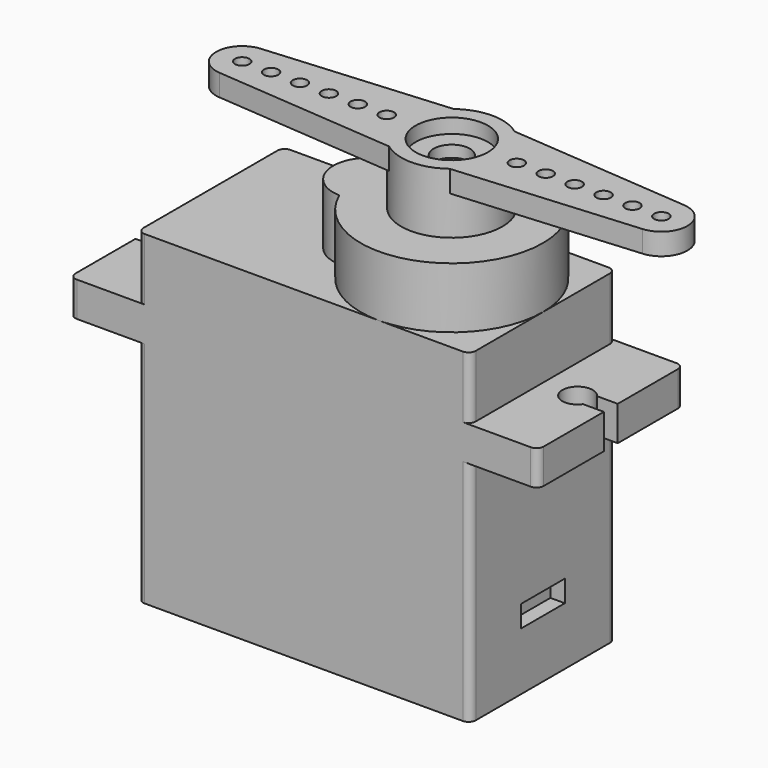
from build123d import *

# Parameters (mm, degrees)
F0_W      = 4.7
F0_H      = 2.4
F1_DEPTH  = 12.6
F3_DEPTH  = 4.2
F4_R      = 2.3
F4_R_2    = 0.9
F5_DEPTH  = 2.5
F7_DEPTH  = 25
F8_R      = 0.5
F9_W      = 3.8
F9_H      = 1.5
F10_DEPTH = 1
F12_R     = 0.5
F13_DEPTH = 1.5
F14_R     = 3.5
F15_DEPTH = 2.7
F16_R     = 2.25
F17_DEPTH = 2.4
F18_R     = 2.5
F19_DEPTH = 1
F20_R     = 1.25
F21_DEPTH = 25


with BuildPart() as f1:
    # F0 (on Front) → F1 (new body)
    with BuildSketch(Plane.XZ):
        Polygon((0, 15.8), (0, 0), (23, 0), (23, 15.8), (23, 18.2), (23, 22.5), (0, 22.5), (0, 18.2), align=None)
        with Locations((-2.35, 17)):
            Rectangle(F0_W, F0_H)
        with Locations((25.35, 17)):
            Rectangle(F0_W, F0_H)
    extrude(amount=F1_DEPTH)

    # F2 (on face) → F3 (join)
    with BuildSketch(Plane.XY.offset(22.5)):
        with BuildLine():
            ThreePointArc((10.9166666667, -3.8013892749), (8.5, -6.3), (10.9166666667, -8.7986107251))
            ThreePointArc((10.9166666667, -8.7986107251), (23, -6.3), (10.9166666667, -3.8013892749))
        make_face()
    extrude(amount=F3_DEPTH)

    # F4 (on face) → F5 (join)
    with BuildSketch(Plane.XY.offset(26.7)):
        with Locations((16.7, -6.3)):
            Circle(F4_R)
        with Locations((16.7, -6.3)):
            Circle(F4_R_2, mode=Mode.SUBTRACT)
    extrude(amount=F5_DEPTH)

    # F6 (on face) → F7 (cut)
    with BuildSketch(Plane.XY.offset(18.2)):
        with BuildLine():
            Line((-5.3876070306, -6.9), (-3.261684397, -6.9))
            ThreePointArc((-3.261684397, -6.9), (-1.35, -6.3), (-3.261684397, -5.7))
            Line((-3.261684397, -5.7), (-5.3876070306, -5.7))
            Line((-5.3876070306, -5.7), (-5.3876070306, -6.9))
        make_face()
        with BuildLine():
            ThreePointArc((26.261684397, -5.7), (24.35, -6.3), (26.261684397, -6.9))
            Line((26.261684397, -6.9), (28.3876070306, -6.9))
            Line((28.3876070306, -6.9), (28.3876070306, -5.7))
            Line((28.3876070306, -5.7), (26.261684397, -5.7))
        make_face()
    extrude(amount=-F7_DEPTH, mode=Mode.SUBTRACT)

    # F8
    f8_edges = [f1.edges().sort_by_distance(p)[0] for p in [
        (0, -12.6, 20.35),
        (0, -12.6, 7.9),
        (0, 0, 20.35),
        (0, 0, 7.9),
        (-4.7, -12.6, 17),
        (-4.7, 0, 17),
        (27.7, -12.6, 17),
        (23, -12.6, 20.35),
        (23, -12.6, 7.9),
        (27.7, 0, 17),
        (23, 0, 20.35),
        (23, 0, 7.9),
    ]]
    fillet(f8_edges, radius=F8_R)

    # F9 (on face) → F10 (cut)
    with BuildSketch(Plane.YZ.offset(23)):
        with Locations((-6.3, 4.75)):
            Rectangle(F9_W, F9_H)
    extrude(amount=-F10_DEPTH, mode=Mode.SUBTRACT)


with BuildPart() as f13:
    # F12 (on offset) → F13 (new body)
    with BuildSketch(Plane(origin=(0, 0, 31), x_dir=(1, 0, 0), z_dir=(0, 0, -1))):
        with BuildLine():
            Line((2.0561389261, 4.5057581012), (14.6, 3.5))
            ThreePointArc((14.6, 3.5), (16.7, 2.8), (18.8, 3.5))
            Line((18.8, 3.5), (31.3438610739, 4.5057581012))
            ThreePointArc((31.3438610739, 4.5057581012), (33, 6.3), (31.3438610739, 8.0942418988))
            Line((31.3438610739, 8.0942418988), (18.8, 9.1))
            ThreePointArc((18.8, 9.1), (16.7, 9.8), (14.6, 9.1))
            Line((14.6, 9.1), (2.0561389261, 8.0942418988))
            ThreePointArc((2.0561389261, 8.0942418988), (0.4, 6.3), (2.0561389261, 4.5057581012))
        make_face()
        with Locations((2.2, 6.3)):
            Circle(F12_R, mode=Mode.SUBTRACT)
        with Locations((4.2, 6.3)):
            Circle(F12_R, mode=Mode.SUBTRACT)
        with Locations((6.2, 6.3)):
            Circle(F12_R, mode=Mode.SUBTRACT)
        with Locations((8.2, 6.3)):
            Circle(F12_R, mode=Mode.SUBTRACT)
        with Locations((10.2, 6.3)):
            Circle(F12_R, mode=Mode.SUBTRACT)
        with Locations((12.2, 6.3)):
            Circle(F12_R, mode=Mode.SUBTRACT)
        with Locations((21.2, 6.3)):
            Circle(F12_R, mode=Mode.SUBTRACT)
        with Locations((23.2, 6.3)):
            Circle(F12_R, mode=Mode.SUBTRACT)
        with Locations((25.2, 6.3)):
            Circle(F12_R, mode=Mode.SUBTRACT)
        with Locations((27.2, 6.3)):
            Circle(F12_R, mode=Mode.SUBTRACT)
        with Locations((29.2, 6.3)):
            Circle(F12_R, mode=Mode.SUBTRACT)
        with Locations((31.2, 6.3)):
            Circle(F12_R, mode=Mode.SUBTRACT)
    extrude(amount=F13_DEPTH)

    # F14 (on face) → F15 (join)
    with BuildSketch(Plane(origin=(0, 0, 29.5), x_dir=(1, 0, 0), z_dir=(0, 0, -1))):
        with Locations((16.7, 6.3)):
            Circle(F14_R)
    extrude(amount=F15_DEPTH)

    # F16 (on face) → F17 (cut)
    with BuildSketch(Plane(origin=(0, 0, 26.8), x_dir=(1, 0, 0), z_dir=(0, 0, -1))):
        with Locations((16.7, 6.3)):
            Circle(F16_R)
    extrude(amount=-F17_DEPTH, mode=Mode.SUBTRACT)

    # F18 (on face) → F19 (cut)
    with BuildSketch(Plane.XY.offset(31)):
        with Locations((16.7, -6.3)):
            Circle(F18_R)
    extrude(amount=-F19_DEPTH, mode=Mode.SUBTRACT)

    # F20 (on face) → F21 (cut)
    with BuildSketch(Plane.XY.offset(30)):
        with Locations((16.7, -6.3)):
            Circle(F20_R)
    extrude(amount=-F21_DEPTH, mode=Mode.SUBTRACT)


solid = Compound([f1.part, f13.part])
